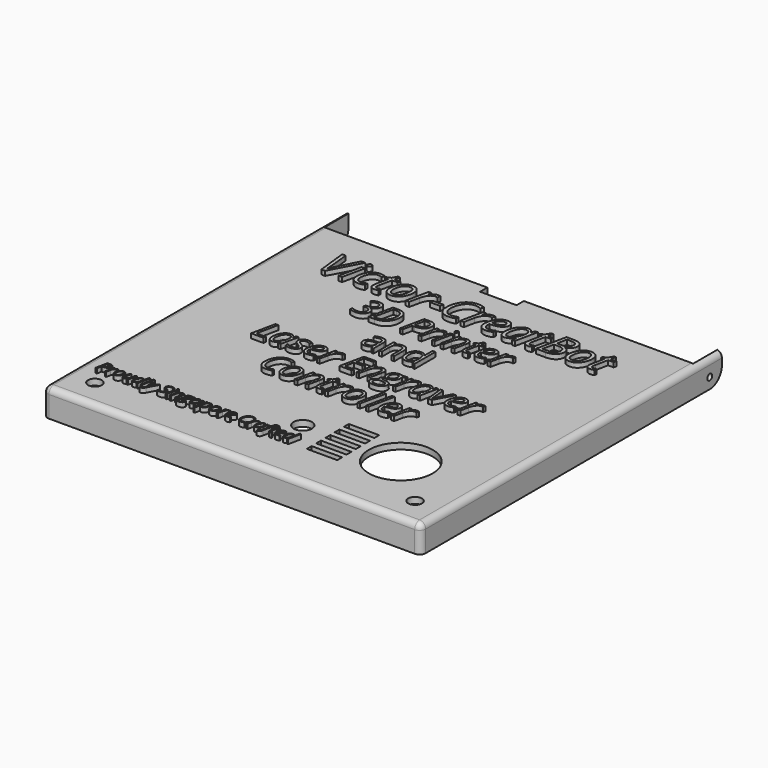
from build123d import *

# Parameters (mm, degrees)
F0_W           = 112.25
F0_H           = 107.75
F0_R           = 2.25
F0_W_2         = 10
F0_H_2         = 2
F0_R_2         = 3
F0_R_3         = 10.5
F1_DEPTH       = 2
F2_W           = 12
F2_H           = 6
F3_DEPTH       = 2.001
F4_DEPTH       = 6
F5_DEPTH       = 6
F6_DEPTH       = 6
F8_DEPTH       = 7
F9_TEXT_SIZE   = 13.8888888889
F9_TEXT_SIZE_2 = 11.1111111111
F9_TEXT_SIZE_3 = 5.5555555556
F10_DEPTH      = 1.5
F12_DEPTH      = 10
F14_DEPTH      = 10
F16_R          = 2
F15_W          = 20
F15_H          = 2
F17_DEPTH      = 2
F18_R          = 0.99999
F19_R          = 1
F20_DEPTH      = 124.251
F21_R          = 5


# Not quite as in the source:
# - a fillet or chamfer is up to 0.001 mm smaller than in the source, because OpenCascade refuses the exact size
# - a feature names something its author has since deleted; it is built from what else it names
# - Text() gives the source's letters only with a copy of the font that has no kerning and outlines rounded to 1/6400 em; it was checked with that copy


with BuildPart() as f1:
    # F0 (on Top) → F1 (new body)
    with BuildSketch(Plane.XY):
        with Locations((56.125, 53.875)):
            Rectangle(F0_W, F0_H)
        with Locations((3.5, 3.5)):
            Circle(F0_R, mode=Mode.SUBTRACT)
        with Locations((74, 9.7260005832)):
            Rectangle(F0_W_2, F0_H_2, mode=Mode.SUBTRACT)
        with Locations((60, 18.3)):
            Circle(F0_R_2, mode=Mode.SUBTRACT)
        with Locations((73.9335712552, 13.6173337221)):
            Rectangle(F0_W_2, F0_H_2, mode=Mode.SUBTRACT)
        with Locations((73.8671425104, 17.5086668611)):
            Rectangle(F0_W_2, F0_H_2, mode=Mode.SUBTRACT)
        with Locations((73.8007137656, 21.4)):
            Rectangle(F0_W_2, F0_H_2, mode=Mode.SUBTRACT)
        with Locations((73.7342850208, 25.2913331389)):
            Rectangle(F0_W_2, F0_H_2, mode=Mode.SUBTRACT)
        with Locations((108.75, 3.5)):
            Circle(F0_R, mode=Mode.SUBTRACT)
        with Locations((92.23, 18.3)):
            Circle(F0_R_3, mode=Mode.SUBTRACT)
    extrude(amount=F1_DEPTH)

    # F2 (on face) → F3 (cut, through all)
    with BuildSketch(Plane.XY.offset(2)):
        with Locations((55.13, 107.75)):
            Rectangle(F2_W, F2_H)
    extrude(amount=-F3_DEPTH, mode=Mode.SUBTRACT)

    # F4 (add): faces of the model
    f4_faces = [f1.faces().sort_by_distance(p)[0] for p in [
        (56.125, 0, 1),
        (56.125, 0, 1),
    ]]
    extrude(f4_faces, amount=F4_DEPTH)

    # F5 (add): faces of the model
    f5_faces = [f1.faces().sort_by_distance(p)[0] for p in [
        (0, 50.875, 1),
        (0, 50.875, 1),
    ]]
    extrude(f5_faces, amount=F5_DEPTH)

    # F6 (add): faces of the model
    f6_faces = [f1.faces().sort_by_distance(p)[0] for p in [
        (112.25, 50.875, 1),
        (112.25, 50.875, 1),
    ]]
    extrude(f6_faces, amount=F6_DEPTH)

    # F7 (on face) → F8 (join)
    with BuildSketch(Plane(origin=(0, 0, 0), x_dir=(1, 0, 0), z_dir=(0, 0, -1))):
        Polygon((116.75, -107.75), (118.25, -107.75), (118.25, 6), (116.75, 6), (61.13, 6), (-4.5, 6), (-6, 6), (-6, -107.75), (-4.5, -107.75), (-4.5, -58.87), (-4.5, 4.5), (61.13, 4.5), (116.75, 4.5), (116.75, -58.87), align=None)
    extrude(amount=F8_DEPTH)

    # F9 (on face) → F10 (join)
    with BuildSketch(Plane.XY.offset(2)):
        with Locations((9, 86.75)):
            Text('Victor-CreatBot', F9_TEXT_SIZE, font='Open Sans', font_style=FontStyle.ITALIC, text_align=(TextAlign.LEFT, TextAlign.BOTTOM))
        with Locations((30.7, 73.75)):
            Text('3D Printer', F9_TEXT_SIZE_2, font='Open Sans', font_style=FontStyle.ITALIC, text_align=(TextAlign.LEFT, TextAlign.BOTTOM))
        with Locations((44, 60.75)):
            Text('and', F9_TEXT_SIZE_2, font='Open Sans', text_align=(TextAlign.LEFT, TextAlign.BOTTOM))
        with Locations((19, 47.75)):
            Text('Laser Engraver', F9_TEXT_SIZE_2, font='Open Sans', font_style=FontStyle.ITALIC, text_align=(TextAlign.LEFT, TextAlign.BOTTOM))
        with Locations((31.1, 34.75)):
            Text('Controller', F9_TEXT_SIZE_2, font='Open Sans', font_style=FontStyle.ITALIC, text_align=(TextAlign.LEFT, TextAlign.BOTTOM))
        with Locations((0, 7.7912404239)):
            Text('Proudly Singapore Crafted', F9_TEXT_SIZE_3, font='Open Sans', font_style=FontStyle.ITALIC, text_align=(TextAlign.LEFT, TextAlign.BOTTOM))
    extrude(amount=F10_DEPTH)

    # F11 (on face) → F12 (join)
    with BuildSketch(Plane(origin=(0, 107.75, 0), x_dir=(-1, 0, 0), z_dir=(0, 1, 0))):
        Polygon((6, -7), (6, 2), (4.5, 2), (4.5, 0), (4.5, -7), align=None)
    extrude(amount=F12_DEPTH)

    # F13 (on face) → F14 (join)
    with BuildSketch(Plane(origin=(0, 107.75, 0), x_dir=(-1, 0, 0), z_dir=(0, 1, 0))):
        Polygon((-116.75, 2), (-118.25, 2), (-118.25, -7), (-116.75, -7), (-116.75, 0), align=None)
    extrude(amount=F14_DEPTH)

    # F16
    f16_edges = [f1.edges().sort_by_distance(p)[0] for p in [
        (-6, -6, -2.5),
        (118.25, -6, -2.5),
        (56.125, -6, 2),
        (118.25, 55.875, 2),
        (-6, 55.875, 2),
    ]]
    fillet(f16_edges, radius=F16_R)

    # F15 (on face) → F17 (join)
    with BuildSketch(Plane(origin=(0, -4.5, 0), x_dir=(-1, 0, 0), z_dir=(0, 1, 0))):
        with Locations((-102.8067821264, -6)):
            Rectangle(F15_W, F15_H)
        with Locations((-10, -6)):
            Rectangle(F15_W, F15_H)
    extrude(amount=F17_DEPTH)

    # F18 (radius 1 in the source; OpenCascade refuses exactly that, so slightly less here)
    f18_edges = [f1.edges().sort_by_distance(p)[0] for p in [
        (102.806782, -2.5, -5),
        (102.806782, -2.5, -7),
        (10, -2.5, -5),
        (10, -2.5, -7),
    ]]
    fillet(f18_edges, radius=F18_R)

    # F19 (on face) → F20 (cut, through all)
    with BuildSketch(Plane(origin=(-6, 0, 0), x_dir=(0, -1, 0), z_dir=(-1, 0, 0))):
        with Locations((-112.75, -3.5)):
            Circle(F19_R)
    extrude(amount=-F20_DEPTH, mode=Mode.SUBTRACT)

    # F21
    f21_edges = [f1.edges().sort_by_distance(p)[0] for p in [
        (-5.25, 117.75, -7),
        (117.5, 117.75, -7),
    ]]
    fillet(f21_edges, radius=F21_R)


solid = f1.part
